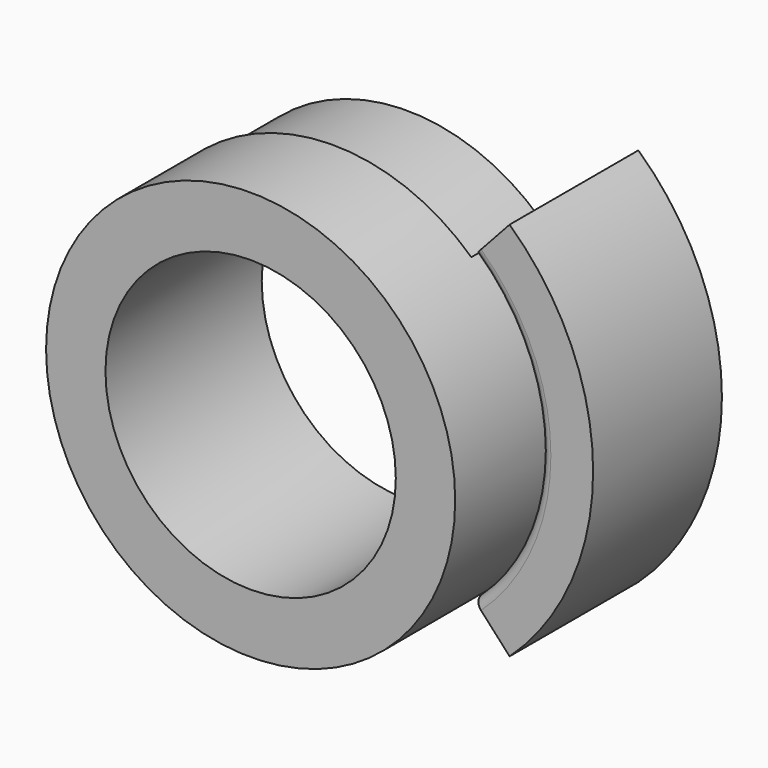
from build123d import *

# Parameters (mm, degrees)
F0_R        = 38.75
F0_R_2      = 27.5
F1_DEPTH    = 37
F5_DEPTH    = 31
F6_T2_ANGLE = 109.624690457
F6_T4_ANGLE = 94.8797670977


# Not quite as in the source:
# - a fillet or chamfer that OpenCascade refuses, or shapes differently, is made with other operations: its cross-section is extruded or revolved along the edge and cut away or added


with BuildPart() as f1:
    # F0 (on Front) → F1 (new body)
    with BuildSketch(Plane.XZ):
        Circle(F0_R)
        Circle(F0_R_2, mode=Mode.SUBTRACT)
    extrude(amount=-F1_DEPTH)

    # F2 (on Right) → F3 (revolve)
    with BuildSketch(Plane.YZ):
        Polygon((20, 48.8753190637), (20, 38.8753190637), (37, 38.8753190637), (37, 37.3753190637), (50.5, 37.3753190637), (50.5, 48.8753190637), align=None)
    revolve(axis=Axis((0, 37, 0), (0, -1, 0)))

    # F4 (on face) → F5 (cut)
    with BuildSketch(Plane(origin=(0, 50.5, 0), x_dir=(-1, 0, 0), z_dir=(0, 1, 0))):
        with BuildLine():
            ThreePointArc((37.3753190637, 0), (15.0348368547, -34.2179507841), (-25.2792982183, -27.5294670617))
            Line((-25.2792982183, -27.5294670617), (-33.057477423, -36))
            ThreePointArc((-33.057477423, -36), (19.6609010104, -44.7464611454), (48.8753190637, 0))
            ThreePointArc((48.8753190637, 0), (19.6609010104, 44.7464611454), (-33.057477423, 36))
            Line((-33.057477423, 36), (-25.2792982183, 27.5294670617))
            ThreePointArc((-25.2792982183, 27.5294670617), (15.0348368547, 34.2179507841), (37.3753190637, 0))
        make_face()
    extrude(amount=-F5_DEPTH, mode=Mode.SUBTRACT)

    # F6: fillet of radius 2 on 2 edges, made by hand

    # F6_s1 → F6_t2 (revolve, cut)
    with BuildSketch(Plane(origin=(0, 0, 0), x_dir=(0, 1, 0), z_dir=(-0.8172690803, 0, -0.5762562368))):
        with BuildLine():
            ThreePointArc((20, 40.8753190637), (20.5857864376, 39.4611055013), (22, 38.8753190637))
            Line((22, 38.8753190637), (20, 38.8753190637))
            Line((20, 38.8753190637), (20, 40.8753190637))
        make_face()
    revolve(axis=Axis((0, 20, 0), (0, -1, 0)), revolution_arc=F6_T2_ANGLE, mode=Mode.SUBTRACT)

    # F6_s3 → F6_t4 (revolve)
    with BuildSketch(Plane(origin=(0, 0, 0), x_dir=(0, 1, 0), z_dir=(-0.7365680816, 0, -0.6763634091))):
        with BuildLine():
            ThreePointArc((39, 37.3753190637), (37.5857864376, 36.789532626), (37, 35.3753190637))
            Line((37, 35.3753190637), (37, 37.3753190637))
            Line((37, 37.3753190637), (39, 37.3753190637))
        make_face()
    revolve(axis=Axis((0, 37, 0), (0, -1, 0)), revolution_arc=F6_T4_ANGLE)


solid = f1.part
